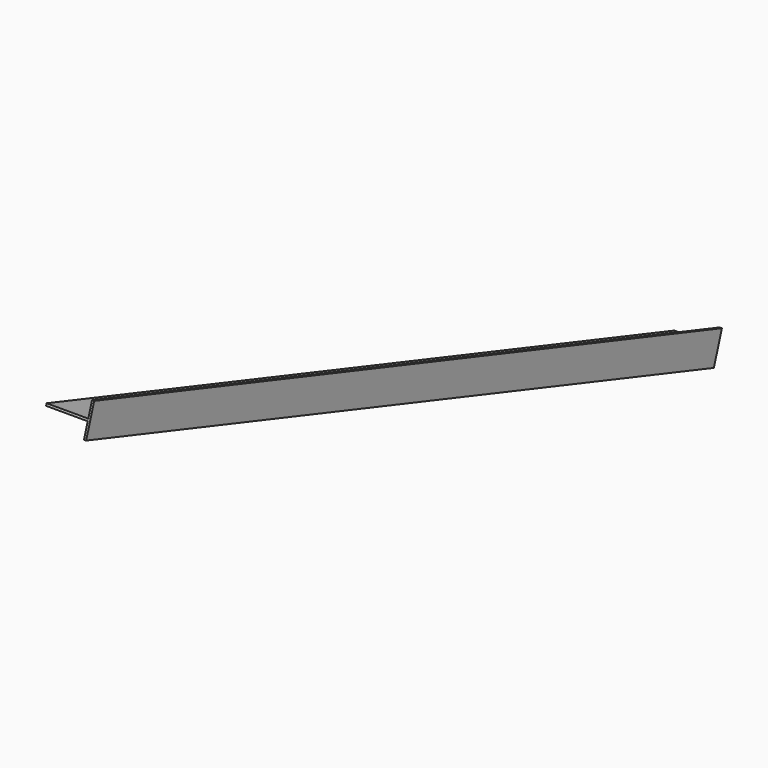
from build123d import *

# Parameters (mm, degrees)
F1_DEPTH = 3
F3_DEPTH = 1143.9908999712


# Not quite as in the source:
# - ends of sketch curves that miss each other by under 0.0002 mm in the source are joined
# - a feature names something its author has since deleted; it is built from what else it names


with BuildPart() as f1:
    # F0 (on Right) → F1 (new body)
    with BuildSketch(Plane.YZ):
        Polygon((-1080.583592135, 376.3379858925), (7.416407865, 22.8253563911), (13.9057647469, 42.7975432333), (-1074.0942352531, 396.3101727347), align=None)
        Polygon((-1088, 353.5126295014), (0, 0), (6.4893568819, 19.9721868422), (-1081.5106431181, 373.4848163436), align=None)
        Polygon((-1081.5106431181, 373.4848163436), (6.4893568819, 19.9721868422), (6.9528823734, 21.3987716166), (-1081.0471176266, 374.911401118), align=None)
        Polygon((-1081.0471176266, 374.911401118), (6.9528823734, 21.3987716166), (7.416407865, 22.8253563911), (-1080.583592135, 376.3379858925), align=None)
    extrude(amount=-F1_DEPTH)

    # F2 (on face) → F3 (join, through all)
    with BuildSketch(Plane(origin=(0, -1088, 353.5126295014), x_dir=(1, 0, 0), z_dir=(0, -0.9510565163, 0.3090169944))):
        Polygon((-60.7660203681, 22.5), (-57.3180156743, 22.5), (-3, 22.5), (-3, 24), (-60.7660203681, 24), align=None)
        Polygon((-3, 21), (-3, 22.5), (-3.1967548982, 21), align=None)
        Polygon((-3.1967548982, 21), (-3, 22.5), (-6.2963244545, 21), align=None)
        Polygon((-3, 22.5), (-57.3180188703, 22.5), (-57.5147689745, 21), (-6.2963244545, 21), align=None)
        Polygon((-57.5147689745, 21), (-57.3180140763, 22.5), (-60.7660203681, 22.5), (-60.7660203681, 21), align=None)
    extrude(amount=-F3_DEPTH)


solid = f1.part
